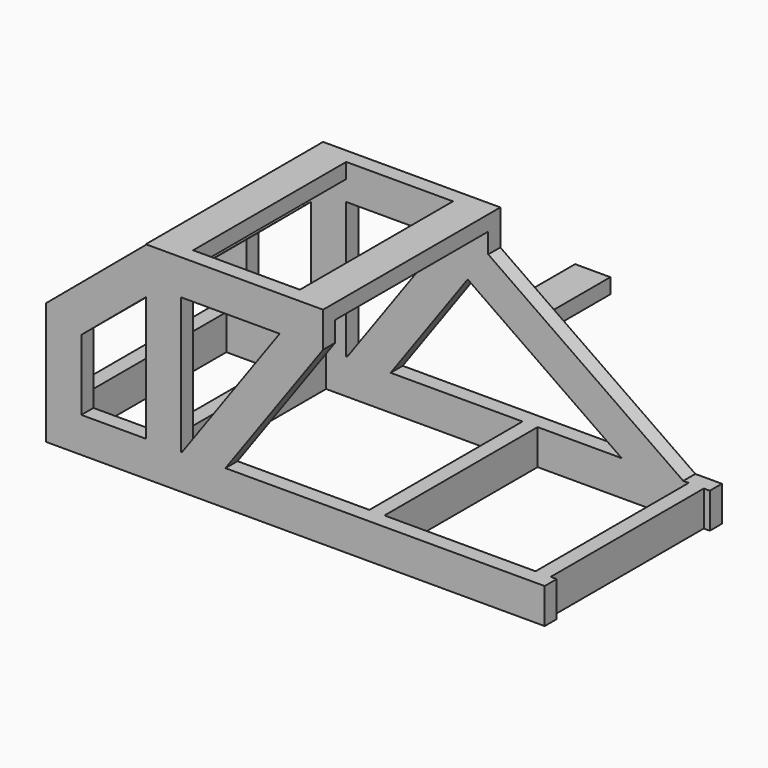
from build123d import *

# Parameters (mm, degrees)
F1_DEPTH = 38.1
F4_W     = 38.1
F4_H     = 88.9
F4_W_2   = 88.9
F4_H_2   = 38.1
F5_DEPTH = 482.6
F7_DEPTH = 38.1
F8_W     = 88.9
F8_H     = 38.1
F9_DEPTH = 177.8


# Not quite as in the source:
# - a feature names something its author has since deleted; it is built from what else it names


with BuildPart() as f1:
    # F0 (on Front) → F1 (new body)
    with BuildSketch(Plane.XZ):
        Polygon((251.46, 403.1040360442), (251.46, 88.9), (340.36, 88.9), (340.36, 431.8), (340.36, 520.7), (251.46, 520.7), (251.46, 519.1547440658), align=None)
        Polygon((0, 308.15475081), (0, 88.9), (88.9, 88.9), (88.9, 266.7), (251.46, 403.1040360442), (251.46, 519.1547440658), align=None)
        Polygon((0, 88.9), (0, 0), (1257.3, 0), (1257.3, 88.9), (452.2981294842, 88.9), (342.8563937201, 88.9), (340.36, 88.9), (251.46, 88.9), (88.9, 88.9), align=None)
        Polygon((673.1, 431.8), (698.5, 431.8), (698.5, 520.7), (340.36, 520.7), (340.36, 431.8), (589.0582642359, 431.8), align=None)
        Polygon((342.8563937201, 88.9), (452.2981294842, 88.9), (698.5, 431.8), (673.1, 431.8), (589.0582642359, 431.8), align=None)
    extrude(amount=-F1_DEPTH)


with BuildPart() as f3_1:
    # F3: instance of F1
    add(f1.part.mirror(Plane(origin=(466.9868832569, 279.4, 206.694910325), x_dir=(1, 0, 0), z_dir=(0, 1, 0))))


with BuildPart() as f1_1:
    add(f1.part)

    add(f3_1.part)  # F5 merges F3_1
    # F4 (on face) → F5 (join, through all)
    with BuildSketch(Plane(origin=(0, 38.1, 0), x_dir=(-1, 0, 0), z_dir=(0, 1, 0))):
        with Locations((-19.05, 44.45)):
            Rectangle(F4_W, F4_H)
        with Locations((-270.51, 44.45)):
            Rectangle(F4_W, F4_H)
        Polygon((-88.9, 266.7), (-31.7561814989, 334.8013509933), (-60.9424747817, 359.2915589223), (-118.0862932828, 291.1902079291), align=None)
        Polygon((-205.6451731313, 364.6608317162), (-148.5013546302, 432.7621827095), (-177.687647913, 457.2523906386), (-234.8314664142, 389.1510396453), align=None)
        with Locations((-803.91, 44.45)):
            Rectangle(F4_W, F4_H)
        Polygon((-251.46, 482.6), (-251.46, 519.1547440658), (-251.46, 520.7), (-340.36, 520.7), (-340.36, 482.6), align=None)
        with Locations((-1223.01, 44.45)):
            Rectangle(F4_W, F4_H)
        with Locations((-654.05, 501.65)):
            Rectangle(F4_W_2, F4_H_2)
    extrude(amount=F5_DEPTH)

    # F6 (on face) → F7 (join)
    with BuildSketch(Plane(origin=(0, 558.8, 0), x_dir=(-1, 0, 0), z_dir=(0, 1, 0))):
        Polygon((-646.6455672201, 359.5792448815), (-698.5, 431.8), (-1190.2829408646, 88.9), (-1034.85039393, 88.9), align=None)
    extrude(amount=-F7_DEPTH)

    # F8 (on face) → F9 (join)
    with BuildSketch(Plane(origin=(0, 558.8, 0), x_dir=(-1, 0, 0), z_dir=(0, 1, 0))):
        with Locations((-789.2684733582, 318.4677249113)):
            Rectangle(F8_W, F8_H)
    extrude(amount=F9_DEPTH)


solid = f1_1.part
